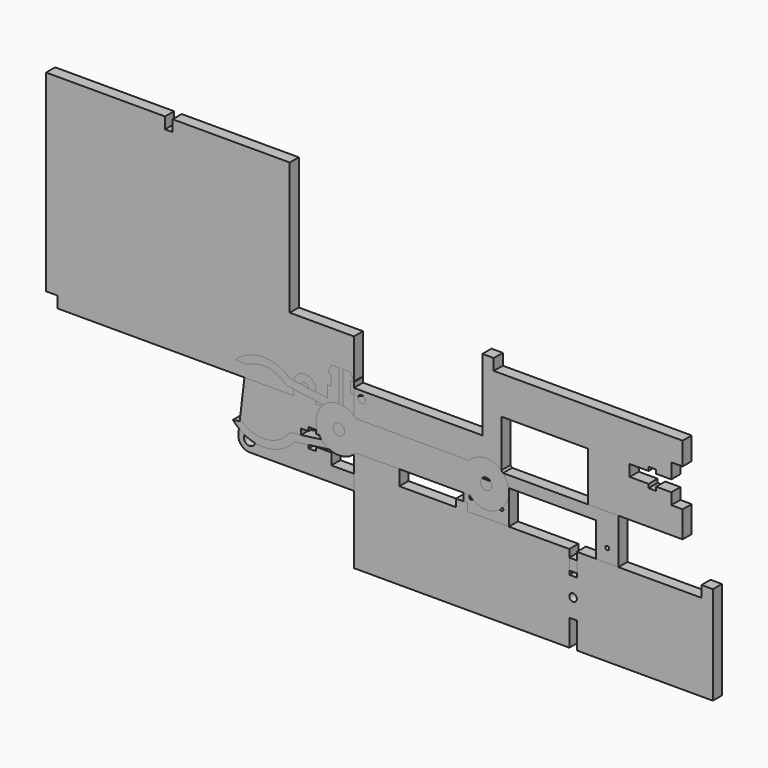
from build123d import *

# Parameters (mm, degrees)
F1_DEPTH  = 3
F2_R      = 0.5
F2_W      = 23
F2_H      = 11
F2_R_2    = 1
F3_DEPTH  = 3
F4_R      = 1
F5_DEPTH  = 3
F6_R      = 1
F7_DEPTH  = 3
F8_R      = 1.5
F8_R_2    = 1
F9_DEPTH  = 3
F10_R     = 1
F10_W     = 4
F10_H     = 2
F11_DEPTH = 3
F13_DEPTH = 3
F14_R     = 1.5
F15_DEPTH = 3


# Not quite as in the source:
# - a feature names something its author has since deleted; it is built from what else it names


with BuildPart() as f1:
    # F0 (on Front) → F1 (new body)
    with BuildSketch(Plane.XZ):
        Polygon((-13.5, 0), (0, 0), (0, 19), (-17, 19), (-17, 54), (-48, 54), (-48, 51), (-50, 51), (-50, 54), (-81.5, 54), (-81.5, 3), (-78.5, 3), (-78.5, 0), (-15.5, 0), (-15.5, 3), (-13.5, 3), align=None)
    extrude(amount=F1_DEPTH)


with BuildPart() as f3:
    # F2 (on Front) → F3 (new body)
    with BuildSketch(Plane.XZ):
        Polygon((34, 0), (0, 0), (0, -17), (34, -17), (34, -14), (36, -14), (36, -17), (70, -17), (70, 0), (36, 0), (36, -3), (34, -3), align=None)
        with Locations((3, -8.5)):
            Circle(F2_R, mode=Mode.SUBTRACT)
        with Locations((17.5, -8.5)):
            Rectangle(F2_W, F2_H, mode=Mode.SUBTRACT)
        with Locations((31, -8.5)):
            Circle(F2_R, mode=Mode.SUBTRACT)
        with Locations((35.026691854, -8.5)):
            Circle(F2_R_2, mode=Mode.SUBTRACT)
        with Locations((39.053383708, -8.5)):
            Circle(F2_R, mode=Mode.SUBTRACT)
        Polygon((41, -14), (41, -3), (41.053383708, -3), (64, -3), (64.053383708, -3), (64.053383708, -14), (64, -14), (41.053383708, -14), align=None, mode=Mode.SUBTRACT)
        with Locations((67.053383708, -8.5)):
            Circle(F2_R, mode=Mode.SUBTRACT)
    extrude(amount=F3_DEPTH)


with BuildPart() as f5:
    # F4 (on Front) → F5 (new body)
    with BuildSketch(Plane.XZ):
        with BuildLine():
            ThreePointArc((0, 3), (0.8786796564, 0.8786796564), (3, 0))
            Line((3, 0), (32, 0))
            ThreePointArc((32, 0), (34.1213203436, 0.8786796564), (35, 3))
            ThreePointArc((35, 3), (34.1213203436, 5.1213203436), (32, 6))
            Line((32, 6), (3, 6))
            ThreePointArc((3, 6), (0.8786796564, 5.1213203436), (0, 3))
        make_face()
        with Locations((3, 3)):
            Circle(F4_R, mode=Mode.SUBTRACT)
        with Locations((32, 3)):
            Circle(F4_R, mode=Mode.SUBTRACT)
    extrude(amount=F5_DEPTH)


with BuildPart() as f7:
    # F6 (on Front) → F7 (new body)
    with BuildSketch(Plane.XZ):
        Polygon((0, 7), (0, 0), (39, 0), (39, 13), (62, 13), (62, 0), (87, 0), (87, 7), (84, 7), (84, 10), (80, 10), (80, 9), (78, 9), (78, 10), (73, 10), (73, 13), (78, 13), (78, 14), (80, 14), (80, 13), (84, 13), (84, 17), (87, 17), (87, 23), (37, 23), (37, 26), (34, 26), (34, 7), align=None)
        with Locations((2.0225740552, 5.0002548265)):
            Circle(F6_R, mode=Mode.SUBTRACT)
    extrude(amount=F7_DEPTH)


with BuildPart() as f9:
    # F8 (on Front) → F9 (new body)
    with BuildSketch(Plane.XZ):
        with BuildLine():
            Line((0, -4), (0, 0))
            Line((0, 0), (-10, 0))
            Line((-10, 0), (-10, 3))
            ThreePointArc((-10, 3), (-10.8786796564, 5.1213203436), (-13, 6))
            ThreePointArc((-13, 6), (-15.1213203436, 5.1213203436), (-16, 3))
            Line((-16, 3), (-16, 0))
            Line((-16, 0), (-29, 0))
            Line((-29, 0), (-30.6058207362, -13.6494762573))
            ThreePointArc((-30.6058207362, -13.6494762573), (-29.8681953246, -15.9935431738), (-27.6263689232, -17))
            Line((-27.6263689232, -17), (0, -17))
            Line((0, -17), (0, -13))
            Line((0, -13), (-6, -13))
            Line((-6, -13), (-6, -10))
            Line((-6, -10), (-10.0000018083, -10))
            Line((-10.0000018083, -10), (-10.0000018083, -11.0026894372))
            Line((-10.0000018083, -11.0026894372), (-12, -11))
            Line((-12, -11), (-12, -10))
            Line((-12, -10), (-14, -10))
            Line((-14, -10), (-14, -7))
            Line((-14, -7), (-12, -7))
            Line((-12, -7), (-12, -6))
            Line((-12, -6), (-10, -6))
            Line((-10, -6), (-10, -7))
            Line((-10, -7), (-6, -7))
            Line((-6, -7), (-6, -4))
            Line((-6, -4), (0, -4))
        make_face()
        with Locations((-27.6263689232, -14)):
            Circle(F8_R, mode=Mode.SUBTRACT)
        with Locations((-13, 3)):
            Circle(F8_R_2, mode=Mode.SUBTRACT)
    extrude(amount=F9_DEPTH)


with BuildPart() as f11:
    # F10 (on Front) → F11 (new body)
    with BuildSketch(Plane.XZ):
        Polygon((12, 0), (0, 0), (0, -35), (57, -35), (57, -28), (59, -28), (59, -35), (95, -35), (95, -9), (92, -9), (92, -12), (59, -12), (59, -18), (57, -18), (57, -12), (30, -12), (30, -10), (27, -10), (27, -12), (12, -12), align=None)
        with Locations((58, -23)):
            Circle(F10_R, mode=Mode.SUBTRACT)
        with Locations((5, -3)):
            Rectangle(F10_W, F10_H, mode=Mode.SUBTRACT)
    extrude(amount=F11_DEPTH)


with BuildPart() as f13:
    # F12 (on Front) → F13 (new body)
    with BuildSketch(Plane.XZ):
        with BuildLine():
            Line((-0.9491760544, 8.4002428828), (0.0508239456, 8.4002428828))
            Line((0.0508239456, 8.4002428828), (-0.9491760544, 10.4002428828))
            Line((-0.9491760544, 10.4002428828), (-2.9491760544, 10.4002428828))
            Line((-2.9491760544, 10.4002428828), (-2.9491760544, -1.5997571172))
            Line((-2.9491760544, -1.5997571172), (-3.9491760544, -1.5997571172))
            Line((-3.9491760544, -1.5997571172), (-3.9491760544, 10.4002428828))
            Line((-3.9491760544, 10.4002428828), (-3.9491760544, 10.4029415973))
            Line((-3.9491760544, 10.4029415973), (-5.9491760544, 10.4029415973))
            Line((-5.9491760544, 10.4029415973), (-6.9491760544, 8.4029415973))
            Line((-6.9491760544, 8.4029415973), (-6.0372303978, 8.4029415973))
            Line((-6.0372303978, 8.4029415973), (-6.0372303978, 5.4029415973))
            Line((-6.0372303978, 5.4029415973), (-7.0372303978, 5.4029415973))
            Line((-7.0372303978, 5.4029415973), (-7.0372303978, 2.396423577))
            Line((-7.0372303978, 2.396423577), (-16.9560426049, 3.6681013667))
            ThreePointArc((-16.9560426049, 3.6681013667), (-24.1489246045, 6.3880111742), (-31.2706908491, 3.4869930119))
            Line((-31.2706908491, 3.4869930119), (-28.4805696202, 3.1292752607))
            ThreePointArc((-28.4805696202, 3.1292752607), (-22.9352548858, 4.3270620373), (-17.8714603281, 1.769095395))
            Line((-17.8714603281, 1.769095395), (-7.0372303978, 0.3800531102))
            Line((-7.0372303978, 0.3800531102), (-7.0372303978, -7.603576423))
            Line((-7.0372303978, -7.603576423), (-16.9986135566, -8.9001505061))
            ThreePointArc((-16.9986135566, -8.9001505061), (-22.9190749769, -12.5328285255), (-29.5721786871, -10.5367263131))
            Line((-29.5721786871, -10.5367263131), (-32.0541233857, -10.8597763475))
            ThreePointArc((-32.0541233857, -10.8597763475), (-23.8942422369, -14.6022225149), (-15.8234885699, -10.6712558493))
            Line((-15.8234885699, -10.6712558493), (0.0508239456, -8.6050546132))
            Line((0.0508239456, -8.6050546132), (0.0508239456, 5.3949453868))
            Line((0.0508239456, 5.3949453868), (-0.9491760544, 5.3949453868))
            Line((-0.9491760544, 5.3949453868), (-0.9491760544, 8.4002428828))
        make_face()
        with BuildLine():
            ThreePointArc((-32.0541233857, -10.8597763475), (-23.8942306495, -14.6032201296), (-15.8234885699, -10.6712558493))
            ThreePointArc((-15.8234885699, -10.6712558493), (-23.8942422369, -14.6022225149), (-32.0541233857, -10.8597763475))
        make_face()
        with BuildLine():
            ThreePointArc((-16.9986135566, -8.9001505061), (-22.9199618583, -12.5260147495), (-29.5721786871, -10.5367263131))
            ThreePointArc((-29.5721786871, -10.5367263131), (-22.9190749769, -12.5328285255), (-16.9986135566, -8.9001505061))
        make_face()
        with BuildLine():
            ThreePointArc((-28.4805696202, 3.1292752607), (-22.9363462684, 4.3185494883), (-17.8714603281, 1.769095395))
            ThreePointArc((-17.8714603281, 1.769095395), (-22.9352548858, 4.3270620373), (-28.4805696202, 3.1292752607))
        make_face()
        with BuildLine():
            ThreePointArc((-16.9560426049, 3.6681013667), (-24.1490159543, 6.3952313837), (-31.2706908491, 3.4869930119))
            ThreePointArc((-31.2706908491, 3.4869930119), (-24.1489246045, 6.3880111742), (-16.9560426049, 3.6681013667))
        make_face()
    extrude(amount=F13_DEPTH)


with BuildPart() as f15:
    # F14 (on Front) → F15 (new body)
    with BuildSketch(Plane.XZ):
        with BuildLine():
            Line((30.527864045, 0), (0.472135955, 0))
            ThreePointArc((0.472135955, 0), (-10, -4), (0.472135955, -8))
            Line((0.472135955, -8), (30.527864045, -8))
            ThreePointArc((30.527864045, -8), (41, -4), (30.527864045, 0))
        make_face()
        with Locations((-4, -4)):
            Circle(F14_R, mode=Mode.SUBTRACT)
        with Locations((35, -4)):
            Circle(F14_R, mode=Mode.SUBTRACT)
    extrude(amount=F15_DEPTH)


solid = Compound([f1.part, f3.part, f5.part, f7.part, f9.part, f11.part, f13.part, f15.part])
